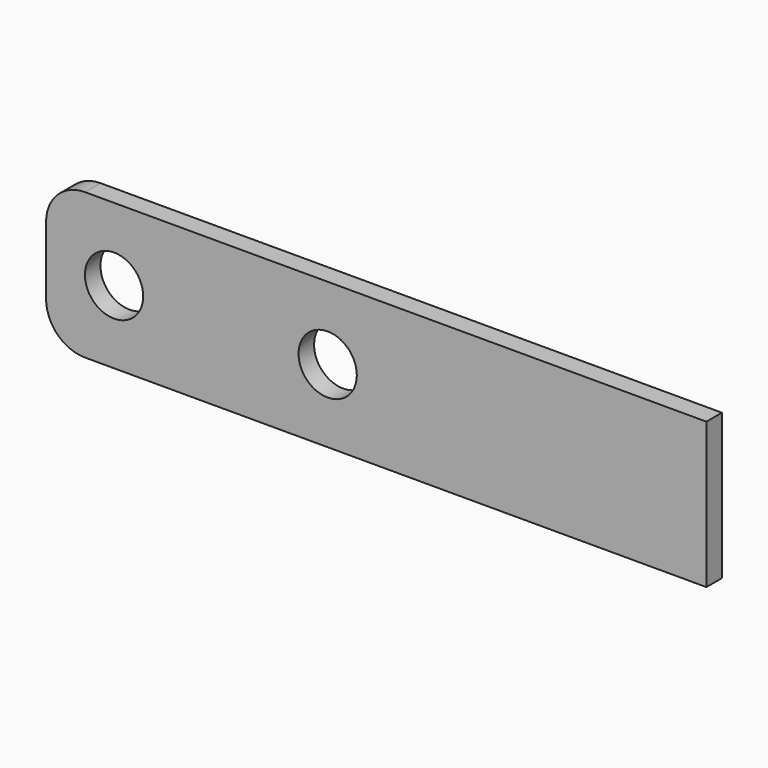
from build123d import *

# Parameters (mm, degrees)
F0_W          = 340
F0_H          = 75
F1_DEPTH      = 10
F2_R          = 20
F3_R          = 15
F4_DEPTH      = 354
F4_DEPTH_BACK = 25


# Not quite as in the source:
# - an extrude ends at something that could not be found from the text; its depth is read off the source's solid


with BuildPart() as f1:
    # F0 (on Front) → F1 (new body)
    with BuildSketch(Plane.XZ):
        Rectangle(F0_W, F0_H)
    extrude(amount=F1_DEPTH)

    # F2
    f2_edges = [f1.edges().sort_by_distance(p)[0] for p in [
        (-170, -5, 37.5),
        (-170, -5, -37.5),
    ]]
    fillet(f2_edges, radius=F2_R)

    # F3 (on Front) → F4 (cut, two sides)
    with BuildSketch(Plane.XZ) as f4_sk:
        with Locations((-135, 0)):
            Circle(F3_R)
        with Locations((-25, 0)):
            Circle(F3_R)
    extrude(amount=-F4_DEPTH, mode=Mode.SUBTRACT)
    extrude(f4_sk.sketch, amount=F4_DEPTH_BACK, mode=Mode.SUBTRACT)


solid = f1.part
